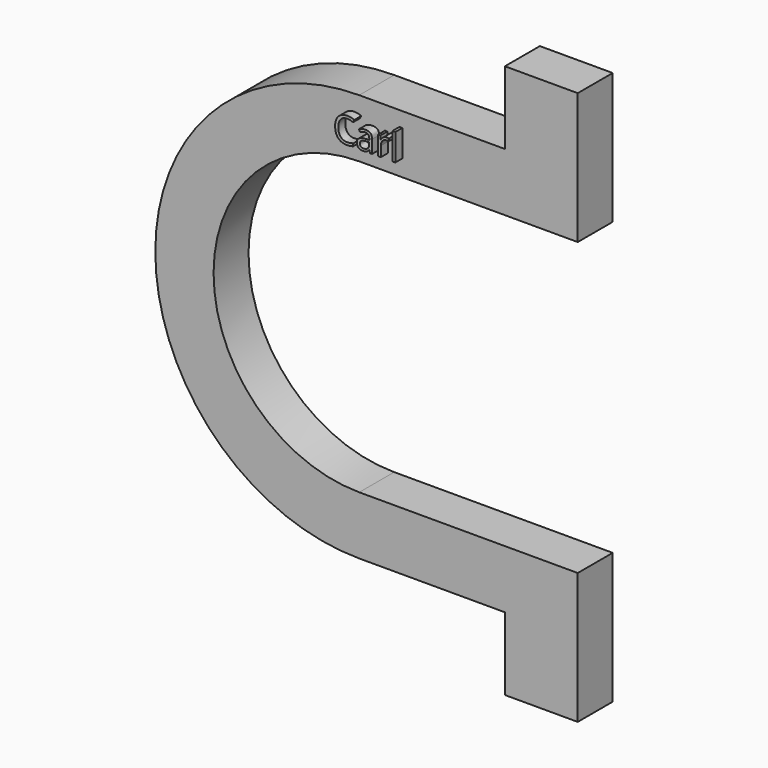
from build123d import *

# Parameters (mm, degrees)
F1_DEPTH     = 38.1
F2_TEXT_SIZE = 30.8327790764
F3_DEPTH     = 45.72


# Not quite as in the source:
# - Text() gives the source's letters only with a copy of the font that has no kerning and outlines rounded to 1/6400 em; it was checked with that copy


with BuildPart() as f1:
    # F0 (on Front) → F1 (new body)
    with BuildSketch(Plane.XZ):
        with BuildLine():
            Line((127, 177.8), (0, 177.8))
            ThreePointArc((0, 177.8), (-125.723585695, 125.723585695), (-177.8, 0))
            ThreePointArc((-177.8, 0), (-125.723585695, -125.723585695), (0, -177.8))
            Line((0, -177.8), (127, -177.8))
            Line((127, -177.8), (127, -241.3))
            Line((127, -241.3), (190.5, -241.3))
            Line((190.5, -241.3), (190.5, -177.8))
            Line((190.5, -177.8), (190.5, -127))
            Line((190.5, -127), (127, -127))
            Line((127, -127), (0, -127))
            ThreePointArc((0, -127), (-127, 0), (0, 127))
            Line((0, 127), (127, 127))
            Line((127, 127), (190.5, 127))
            Line((190.5, 127), (190.5, 177.8))
            Line((190.5, 177.8), (190.5, 241.3))
            Line((190.5, 241.3), (127, 241.3))
            Line((127, 241.3), (127, 177.8))
        make_face()
    extrude(amount=F1_DEPTH)

    # F2 (on Front) → F3 (join)
    with BuildSketch(Plane.XZ):
        with Locations((-16.814801842, 141.401797533)):
            Text('Carl', F2_TEXT_SIZE, font='Open Sans', text_align=(TextAlign.LEFT, TextAlign.BOTTOM))
    extrude(amount=F3_DEPTH)


solid = f1.part
